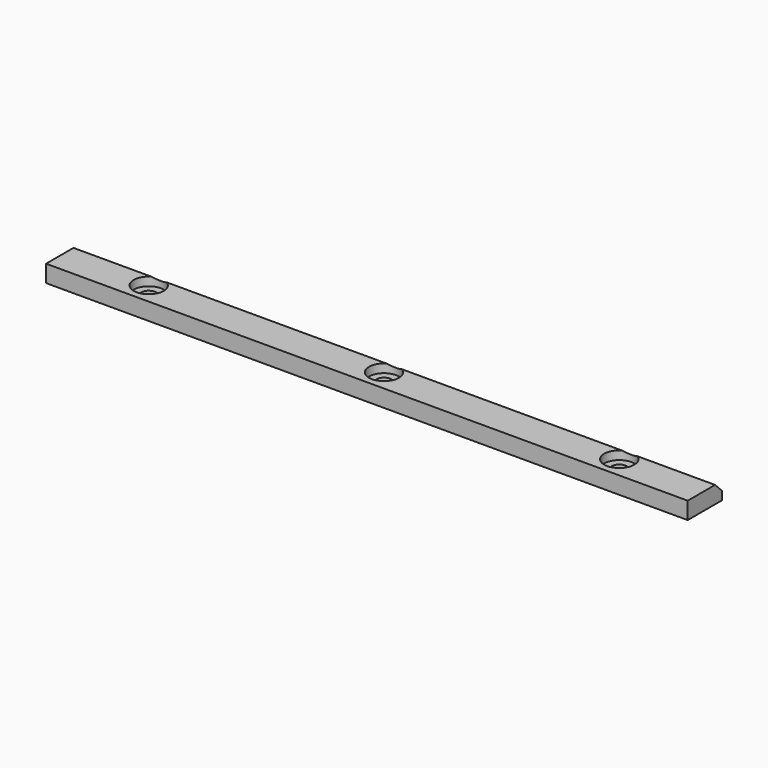
from build123d import *

# Parameters (mm, degrees)
F0_W           = 150
F0_H           = 10
F1_DEPTH       = 4
F2_D           = 3.5
F2_CBORE_D     = 7
F2_CBORE_DEPTH = 2
F3_T1_DEPTH    = 160.2867319519


# Not quite as in the source:
# - a fillet or chamfer that OpenCascade refuses, or shapes differently, is made with other operations: its cross-section is extruded or revolved along the edge and cut away or added


with BuildPart() as f1:
    # F0 (on Top) → F1 (new body)
    with BuildSketch(Plane.XY):
        with Locations((0, 5)):
            Rectangle(F0_W, F0_H)
    extrude(amount=-F1_DEPTH)

    # F2 (through all)
    with Locations(Plane.XY):
        with Locations((-55, 5), (0, 5), (55, 5)):
            CounterBoreHole(F2_D / 2, F2_CBORE_D / 2, F2_CBORE_DEPTH)

    # F3: chamfer of 2 on 1 edges, made by hand

    # F3_s2 → F3_t1 (cut)
    with BuildSketch(Plane.YZ.offset(-80.1433659759)):
        Polygon((10, -2), (8, 0), (10, 0), align=None)
    extrude(amount=F3_T1_DEPTH, mode=Mode.SUBTRACT)


solid = f1.part
